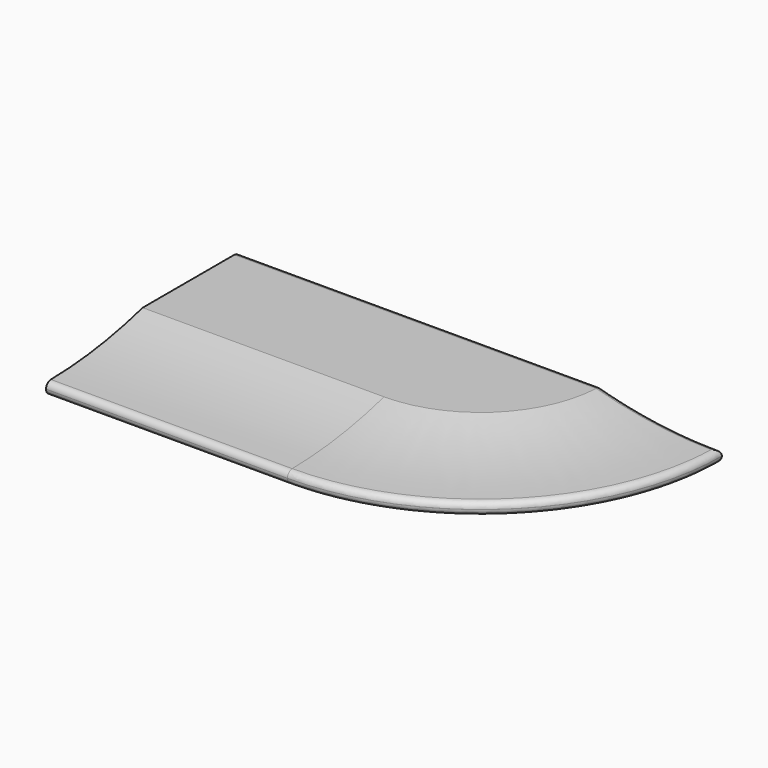
from build123d import *

# Parameters (mm, degrees)
F1_DEPTH = 4.7625
F2_W     = 19.05
F2_H     = 6.35
F3_DEPTH = 25.4
F4_R     = 2.54
F9_R     = 1.26999


# Not quite as in the source:
# - a fillet or chamfer is up to 0.001 mm smaller than in the source, because OpenCascade refuses the exact size


with BuildPart() as f1:
    # F0 (on Top) → F1 (new body, symmetric)
    with BuildSketch(Plane.XY):
        with BuildLine():
            Line((101.6, 0), (0, 0))
            Line((0, 0), (0, -50.8))
            Line((0, -50.8), (50.8, -50.8))
            ThreePointArc((50.8, -50.8), (86.7210244843, -35.9210244843), (101.6, 0))
        make_face()
    extrude(amount=F1_DEPTH, both=True)

    # F2 (on face) → F3 (cut)
    with BuildSketch(Plane(origin=(0, 0, 0), x_dir=(0, -1, 0), z_dir=(-1, 0, 0))):
        with Locations((12.7, 0)):
            Rectangle(F2_W, F2_H)
    extrude(amount=-F3_DEPTH, mode=Mode.SUBTRACT)

    # F4
    f4_edges = [f1.edges().sort_by_distance(p)[0] for p in [
        (12.7, -3.175, 3.175),
        (12.7, -22.225, 3.175),
        (12.7, -3.175, -3.175),
        (12.7, -22.225, -3.175),
    ]]
    fillet(f4_edges, radius=F4_R)


with BuildPart() as f6:
    # F6: sweep along a path in F6_path
    with BuildLine(Plane(origin=(50.8, -50.8, 4.7625), x_dir=(0, 1, 0), z_dir=(0, 0, 1))) as f6_path:
        Line((0, 50.8), (0, 0))
        ThreePointArc((0, 0), (14.8789755157, -35.9210244843), (50.8, -50.8))
    # F5 (on face) → F6 (sweep)
    with BuildSketch(Plane(origin=(0, 0, 0), x_dir=(0, -1, 0), z_dir=(-1, 0, 0))):
        with BuildLine():
            Line((50.8, 4.7625), (25.4, 4.7625))
            ThreePointArc((25.4, 4.7625), (37.9805074569, 2.1472133229), (50.8, 1.27))
            Line((50.8, 1.27), (50.8, 4.7625))
        make_face()
    sweep(path=f6_path.line)


with BuildPart() as f7_1:
    # F7: instance of F6
    add(f6.part.mirror(Plane.XY))


with BuildPart() as f1_1:
    add(f1.part)

    # F8: cut F6, F7_1
    add(f6.part, mode=Mode.SUBTRACT)
    add(f7_1.part, mode=Mode.SUBTRACT)

    # F9 (radius 1.27 in the source; OpenCascade refuses exactly that, so slightly less here)
    f9_edges = [f1_1.edges().sort_by_distance(p)[0] for p in [
        (38.1, 0, 4.7625),
        (38.1, 0, -4.7625),
        (88.780507, 0, 2.147213),
        (88.780507, 0, -2.147213),
        (25.4, -50.8, 1.27),
        (25.4, -50.8, -1.27),
        (86.721024, -35.921024, 1.27),
        (86.721024, -35.921024, -1.27),
    ]]
    fillet(f9_edges, radius=F9_R)


solid = f1_1.part
